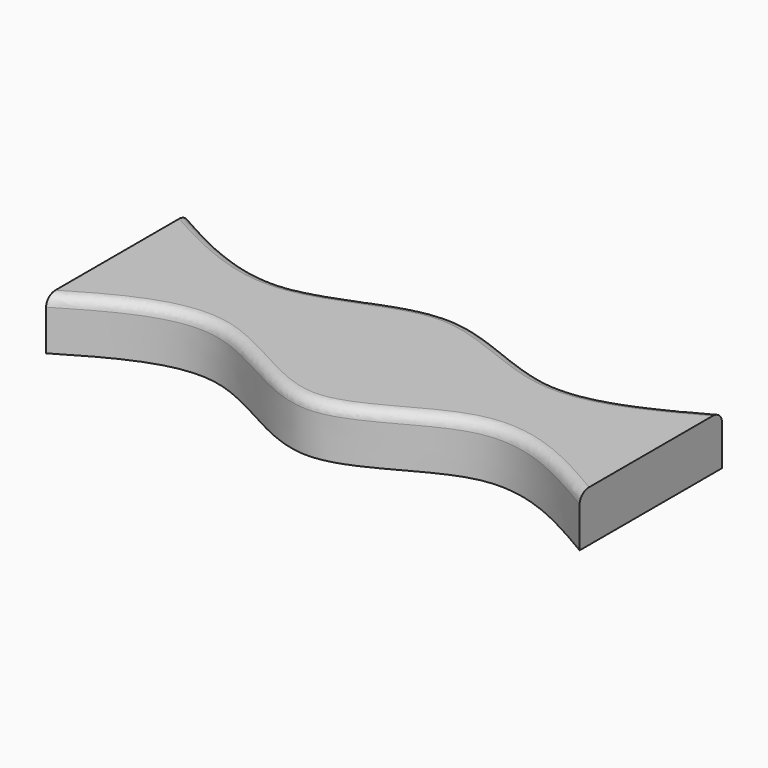
from build123d import *

# Parameters (mm, degrees)
F1_DEPTH = 25.4
F2_R     = 5.08


with BuildPart() as f1:
    # F0 (on Top) → F1 (new body)
    with BuildSketch(Plane.XY):
        with BuildLine():
            Line((-66.675, 0), (0, 0))
            Line((0, 0), (0, 40.6527627649))
            add(Edge.make_bspline(
                [(-66.675, 22.225), (-44.5375090127, 24.3723570613), (-22.2687545064, 40.6527627649), (0, 40.6527627649)],
                knots=[0.2509921979, 0.2509921979, 0.2509921979, 0.2509921979, 0.5, 0.5, 0.5, 0.5], degree=3))
            Line((-66.675, 22.225), (-66.675, 0))
        make_face()
        with BuildLine():
            Line((66.675, 0), (0, 0))
            Line((0, 0), (0, -48.2472372351))
            add(Edge.make_bspline(
                [(0, -48.2472372351), (22.1739498153, -48.2472372351), (44.3478996306, -26.4101755095), (66.675, -22.225)],
                knots=[0.5, 0.5, 0.5, 0.5, 0.7511380765, 0.7511380765, 0.7511380765, 0.7511380765], degree=3))
            Line((66.675, -22.225), (66.675, 0))
        make_face()
        with BuildLine():
            Line((0, -48.2472372351), (0, 0))
            Line((0, 0), (-66.675, 0))
            Line((-66.675, 0), (-66.675, -22.225))
            add(Edge.make_bspline(
                [(-66.675, -22.225), (-44.3478996306, -26.4101755095), (-22.1739498153, -48.2472372351), (0, -48.2472372351)],
                knots=[0.2488619235, 0.2488619235, 0.2488619235, 0.2488619235, 0.5, 0.5, 0.5, 0.5], degree=3))
        make_face()
        with BuildLine():
            Line((0, 40.6527627649), (0, 0))
            Line((0, 0), (66.675, 0))
            Line((66.675, 0), (66.675, 22.225))
            add(Edge.make_bspline(
                [(0, 40.6527627649), (22.2687545064, 40.6527627649), (44.5375090127, 24.3723570613), (66.675, 22.225)],
                knots=[0.5, 0.5, 0.5, 0.5, 0.7490078021, 0.7490078021, 0.7490078021, 0.7490078021], degree=3))
        make_face()
        with BuildLine():
            Line((-66.675, -22.225), (-66.675, 0))
            Line((-66.675, 0), (-133.35, 0))
            Line((-133.35, 0), (-133.35, -44.45))
            add(Edge.make_bspline(
                [(-133.35, -44.45), (-111.0748709935, -31.2638781059), (-88.7997419869, -18.0777562117), (-66.675, -22.225)],
                knots=[0, 0, 0, 0, 0.2488619235, 0.2488619235, 0.2488619235, 0.2488619235], degree=3))
        make_face()
        with BuildLine():
            Line((-133.35, 0), (-66.675, 0))
            Line((-66.675, 0), (-66.675, 22.225))
            add(Edge.make_bspline(
                [(-133.35, 44.45), (-111.1694546629, 32.2552650985), (-88.9889093259, 20.060530197), (-66.675, 22.225)],
                knots=[0, 0, 0, 0, 0.2509921979, 0.2509921979, 0.2509921979, 0.2509921979], degree=3))
            Line((-133.35, 44.45), (-133.35, 0))
        make_face()
        with BuildLine():
            Line((66.675, 22.225), (66.675, 0))
            Line((66.675, 0), (133.35, 0))
            Line((133.35, 0), (133.35, 44.45))
            add(Edge.make_bspline(
                [(66.675, 22.225), (88.9889093259, 20.060530197), (111.1694546629, 32.2552650985), (133.35, 44.45)],
                knots=[0.7490078021, 0.7490078021, 0.7490078021, 0.7490078021, 1, 1, 1, 1], degree=3))
        make_face()
        with BuildLine():
            Line((133.35, 0), (66.675, 0))
            Line((66.675, 0), (66.675, -22.225))
            add(Edge.make_bspline(
                [(66.675, -22.225), (88.7997419869, -18.0777562117), (111.0748709935, -31.2638781059), (133.35, -44.45)],
                knots=[0.7511380765, 0.7511380765, 0.7511380765, 0.7511380765, 1, 1, 1, 1], degree=3))
            Line((133.35, -44.45), (133.35, 0))
        make_face()
    extrude(amount=F1_DEPTH)

    # F2
    f2_edges = [f1.edges().sort_by_distance(p)[0] for p in [
        (0, -48.247237, 25.4),
        (0, 40.652763, 25.4),
    ]]
    fillet(f2_edges, radius=F2_R)


solid = f1.part
